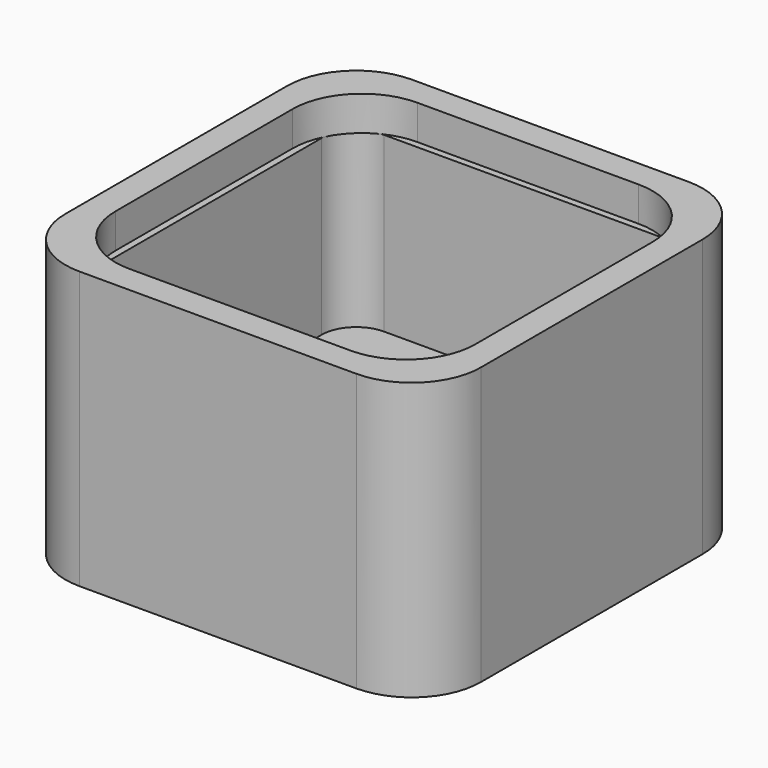
from build123d import *

# Parameters (mm, degrees)
F0_W         = 30
F0_H         = 30
F1_DEPTH     = 20
F2_W         = 25.9800008498
F2_H         = 25.9800008498
F3_DEPTH     = 2.5
F4_W         = 25.9800008498
F4_H         = 25.9800008498
F5_DEPTH     = 2.5
F6_R         = 5
F7_T         = 2.5
F7_T3_DEPTH  = 20.9800008498
F7_T5_DEPTH  = 20.9800008498
F7_T8_ANGLE  = 90.000000001
F7_T10_ANGLE = 90.000000001
F7_T12_ANGLE = 90.000000001
F7_T14_ANGLE = 90.000000001
F8_R         = 1.4393768416
F9_DEPTH     = 25


# Not quite as in the source:
# - a shell that OpenCascade refuses in one call is made with other operations: the cavity is built on its own and cut out


with BuildPart() as f1:
    # F0 (on Top) → F1 (new body)
    with BuildSketch(Plane.XY):
        Rectangle(F0_W, F0_H)
    extrude(amount=F1_DEPTH)

    # F2 (on face) → F3 (cut)
    with BuildSketch(Plane.XY):
        Rectangle(F2_W, F2_H)
    extrude(amount=F3_DEPTH, mode=Mode.SUBTRACT)

    # F4 (on face) → F5 (cut)
    with BuildSketch(Plane.XY.offset(20)):
        Rectangle(F4_W, F4_H)
    extrude(amount=-F5_DEPTH, mode=Mode.SUBTRACT)

    # F6
    f6_edges = [f1.edges().sort_by_distance(p)[0] for p in [
        (-15, -15, 10),
        (-12.99, -12.99, 18.75),
        (-12.99, 12.99, 18.75),
        (12.99, -12.99, 18.75),
        (15, -15, 10),
        (15, 15, 10),
        (-15, 15, 10),
        (12.99, 12.99, 18.75),
        (-12.99, 12.99, 1.25),
        (12.99, -12.99, 1.25),
        (-12.99, -12.99, 1.25),
        (12.99, 12.99, 1.25),
    ]]
    fillet(f6_edges, radius=F6_R)

    # F7: shell of thickness 2.5, made by hand


with BuildPart() as f7_core1:
    # F7_t2: copy of F1
    add(f1.part)

    # the walls: a layer under each face that stays
    f7_faces = [f7_core1.faces().sort_by_distance(p)[0] for p in [
        (0, 15, 10),
        (-12.8571428571, -12.8571428571, 0),
        (13.5355339059, 13.5355339059, 10),
        (-13.5355339059, 13.5355339059, 10),
        (-12.8571428571, -12.8571428571, 20),
        (15, 0, 10),
        (-15, 0, 10),
        (13.5355339059, -13.5355339059, 10),
        (-13.5355339059, -13.5355339059, 10),
        (0, -15, 10),
        (-12.9900004249, 0, 1.25),
        (-11.5255343308, 11.5255343308, 1.25),
        (-11.5255343308, -11.5255343308, 1.25),
        (0, 12.9900004249, 1.25),
        (0, -12.9900004249, 1.25),
        (11.5255343308, 11.5255343308, 1.25),
        (11.5255343308, -11.5255343308, 1.25),
        (12.9900004249, 0, 1.25),
        (0, 12.9900004249, 18.75),
        (11.5255343308, 11.5255343308, 18.75),
        (-11.5255343308, 11.5255343308, 18.75),
        (12.9900004249, 0, 18.75),
        (-12.9900004249, 0, 18.75),
        (11.5255343308, -11.5255343308, 18.75),
        (-11.5255343308, -11.5255343308, 18.75),
        (0, -12.9900004249, 18.75),
        (0, 0, 2.5),
    ]]
    thicken(f7_faces, amount=-F7_T, mode=Mode.SUBTRACT)

    # F7_s4 → F7_t3 (cut)
    with BuildSketch(Plane.XZ.offset(-10.4900004249)):
        Polygon((-12.9650004249, 2.475), (-15.4900004249, 2.5), (-15.4900004249, 5), (-12.9900004249, 5), align=None)
        Polygon((12.9650004249, 2.475), (15.4900004249, 2.5), (15.4900004249, 5), (12.9900004249, 5), align=None)
    extrude(amount=F7_T3_DEPTH, mode=Mode.SUBTRACT)

    # F7_s6 → F7_t5 (cut)
    with BuildSketch(Plane.YZ.offset(-10.4900004249)):
        Polygon((12.9650004249, 2.475), (15.4900004249, 2.5), (15.4900004249, 5), (12.9900004249, 5), align=None)
        Polygon((-12.9650004249, 2.475), (-15.4900004249, 2.5), (-15.4900004249, 5), (-12.9900004249, 5), align=None)
    extrude(amount=F7_T5_DEPTH, mode=Mode.SUBTRACT)

    # F7_s7 → F7_t8 (revolve, cut)
    with BuildSketch(Plane.XZ.offset(-7.9900004249)):
        Polygon((-12.9650004249, 2.475), (-15.4900004249, 2.5), (-15.4900004249, 5), (-12.9900004249, 5), align=None)
    revolve(axis=Axis((-7.9900004249, 7.9900004249, 2.5), (0, 0, -1)), revolution_arc=F7_T8_ANGLE, mode=Mode.SUBTRACT)

    # F7_s9 → F7_t10 (revolve, cut)
    with BuildSketch(Plane.XZ.offset(7.9900004249)):
        Polygon((-12.9650004249, 2.475), (-15.4900004249, 2.5), (-15.4900004249, 5), (-12.9900004249, 5), align=None)
    revolve(axis=Axis((-7.9900004249, -7.9900004249, 2.5), (0, 0, 1)), revolution_arc=F7_T10_ANGLE, mode=Mode.SUBTRACT)

    # F7_s11 → F7_t12 (revolve, cut)
    with BuildSketch(Plane.XZ.offset(-7.9900004249)):
        Polygon((12.9650004249, 2.475), (15.4900004249, 2.5), (15.4900004249, 5), (12.9900004249, 5), align=None)
    revolve(axis=Axis((7.9900004249, 7.9900004249, 2.5), (0, 0, 1)), revolution_arc=F7_T12_ANGLE, mode=Mode.SUBTRACT)

    # F7_s13 → F7_t14 (revolve, cut)
    with BuildSketch(Plane.YZ.offset(7.9900004249)):
        Polygon((-12.9650004249, 2.475), (-15.4900004249, 2.5), (-15.4900004249, 5), (-12.9900004249, 5), align=None)
    revolve(axis=Axis((7.9900004249, -7.9900004249, 2.5), (0, 0, 1)), revolution_arc=F7_T14_ANGLE, mode=Mode.SUBTRACT)


with BuildPart() as f1_1:
    add(f1.part)

    # what is left inside the walls is the cavity
    f7_cavity = [f7_core1.part.solids().sort_by_distance(p)[0] for p in [
        (0, -4.166667, 17.475),
    ]]
    add(f7_cavity, mode=Mode.SUBTRACT)

    # F8 (on face) → F9 (cut)
    with BuildSketch(Plane.XY.offset(5)):
        Circle(F8_R)
        with Locations((0, 7.2)):
            Circle(F8_R)
        with Locations((5.1, 0)):
            Circle(F8_R)
        with Locations((5.1, 7.2)):
            Circle(F8_R)
        with Locations((10.2, 0)):
            Circle(F8_R)
        with Locations((10.2, 7.2)):
            Circle(F8_R)
        with Locations((-5.1, 0)):
            Circle(F8_R)
        with Locations((-10.2, 0)):
            Circle(F8_R)
        with Locations((-10.2, 7.2)):
            Circle(F8_R)
        with Locations((-5.1, 7.2)):
            Circle(F8_R)
    extrude(amount=-F9_DEPTH, mode=Mode.SUBTRACT)


solid = f1_1.part
